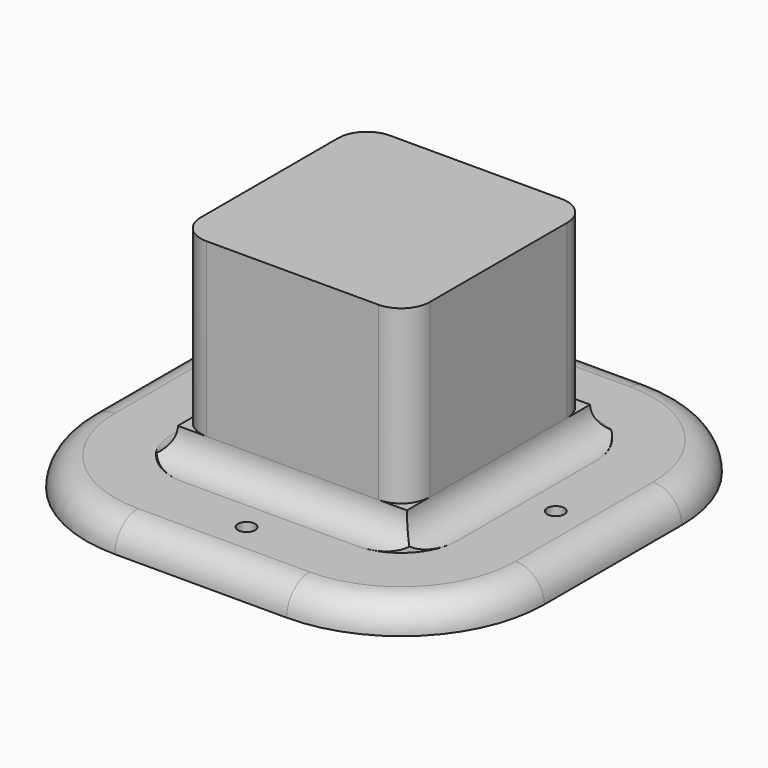
from build123d import *

# Parameters (mm, degrees)
F1_DEPTH  = 40
F0_R      = 1.5
F2_DEPTH  = 5
F3_R      = 4.99999
F4_DEPTH  = 10
F6_DEPTH  = 50
F7_DEPTH  = 5
F8_R      = 5
F9_DEPTH  = 50
F10_DEPTH = 5


# Not quite as in the source:
# - a fillet or chamfer is up to 0.001 mm smaller than in the source, because OpenCascade refuses the exact size


with BuildPart() as f1:
    # F0 (on Top) → F1 (new body)
    with BuildSketch(Plane.XY):
        with BuildLine():
            ThreePointArc((0, 5), (1.464466, 1.464466), (5, 0))
            Line((5, 0), (35, 0))
            ThreePointArc((35, 0), (38.535534, 1.464466), (40, 5))
            Line((40, 5), (40, 35))
            ThreePointArc((40, 35), (38.535534, 38.535534), (35, 40))
            Line((35, 40), (5, 40))
            ThreePointArc((5, 40), (1.464466, 38.535534), (0, 35))
            Line((0, 35), (0, 5))
        make_face()
    extrude(amount=F1_DEPTH)

    # F0 (on Top) → F2 (join)
    with BuildSketch(Plane.XY):
        with BuildLine():
            ThreePointArc((-20, 5), (-12.67767, -12.67767), (5, -20))
            Line((5, -20), (35, -20))
            ThreePointArc((35, -20), (52.67767, -12.67767), (60, 5))
            Line((60, 5), (60, 35))
            ThreePointArc((60, 35), (52.67767, 52.67767), (35, 60))
            Line((35, 60), (5, 60))
            ThreePointArc((5, 60), (-12.67767, 52.67767), (-20, 35))
            Line((-20, 35), (-20, 5))
        make_face()
        with Locations((20, -10)):
            Circle(F0_R, mode=Mode.SUBTRACT)
        with Locations((-10, 20)):
            Circle(F0_R, mode=Mode.SUBTRACT)
        with BuildLine():
            ThreePointArc((-5, 35), (-2.071068, 42.071068), (5, 45))
            Line((5, 45), (35, 45))
            ThreePointArc((35, 45), (42.071068, 42.071068), (45, 35))
            Line((45, 35), (45, 5))
            ThreePointArc((45, 5), (42.071068, -2.071068), (35, -5))
            Line((35, -5), (5, -5))
            ThreePointArc((5, -5), (-2.071068, -2.071068), (-5, 5))
            Line((-5, 5), (-5, 35))
        make_face(mode=Mode.SUBTRACT)
        with Locations((50, 20)):
            Circle(F0_R, mode=Mode.SUBTRACT)
        with Locations((20, 50)):
            Circle(F0_R, mode=Mode.SUBTRACT)
        with BuildLine():
            Line((35, 45), (5, 45))
            ThreePointArc((5, 45), (-2.071068, 42.071068), (-5, 35))
            Line((-5, 35), (-5, 5))
            ThreePointArc((-5, 5), (-2.071068, -2.071068), (5, -5))
            Line((5, -5), (35, -5))
            ThreePointArc((35, -5), (42.071068, -2.071068), (45, 5))
            Line((45, 5), (45, 35))
            ThreePointArc((45, 35), (42.071068, 42.071068), (35, 45))
        make_face()
        with BuildLine():
            Line((35, 0), (5, 0))
            ThreePointArc((5, 0), (1.464466, 1.464466), (0, 5))
            Line((0, 5), (0, 35))
            ThreePointArc((0, 35), (1.464466, 38.535534), (5, 40))
            Line((5, 40), (35, 40))
            ThreePointArc((35, 40), (38.535534, 38.535534), (40, 35))
            Line((40, 35), (40, 5))
            ThreePointArc((40, 5), (38.535534, 1.464466), (35, 0))
        make_face(mode=Mode.SUBTRACT)
    extrude(amount=F2_DEPTH)

    # F3 (radius 5 in the source; OpenCascade refuses exactly that, so slightly less here)
    f3_edges = [f1.edges().sort_by_distance(p)[0] for p in [
        (20, -20, 5),
        (0, 5, 22.5),
    ]]
    fillet(f3_edges, radius=F3_R)

    # F0 (on Top) → F4 (join)
    with BuildSketch(Plane.XY):
        with BuildLine():
            Line((35, 45), (5, 45))
            ThreePointArc((5, 45), (-2.071068, 42.071068), (-5, 35))
            Line((-5, 35), (-5, 5))
            ThreePointArc((-5, 5), (-2.071068, -2.071068), (5, -5))
            Line((5, -5), (35, -5))
            ThreePointArc((35, -5), (42.071068, -2.071068), (45, 5))
            Line((45, 5), (45, 35))
            ThreePointArc((45, 35), (42.071068, 42.071068), (35, 45))
        make_face()
        with BuildLine():
            Line((35, 0), (5, 0))
            ThreePointArc((5, 0), (1.464466, 1.464466), (0, 5))
            Line((0, 5), (0, 35))
            ThreePointArc((0, 35), (1.464466, 38.535534), (5, 40))
            Line((5, 40), (35, 40))
            ThreePointArc((35, 40), (38.535534, 38.535534), (40, 35))
            Line((40, 35), (40, 5))
            ThreePointArc((40, 5), (38.535534, 1.464466), (35, 0))
        make_face(mode=Mode.SUBTRACT)
    extrude(amount=F4_DEPTH)

    # F5 (on face) → F6 (cut)
    with BuildSketch(Plane.XZ.offset(5)):
        with BuildLine():
            ThreePointArc((50, 10), (41.464466, 13.535534), (45, 5))
            ThreePointArc((45, 5), (48.535534, 6.464466), (50, 10))
        make_face()
        with BuildLine():
            ThreePointArc((0, 10), (-8.535534, 13.535534), (-5, 5))
            ThreePointArc((-5, 5), (-1.464466, 6.464466), (0, 10))
        make_face()
    extrude(amount=-F6_DEPTH, mode=Mode.SUBTRACT)

    # F5 (on face) → F7 (cut)
    with BuildSketch(Plane.XZ.offset(5)):
        with BuildLine():
            ThreePointArc((50, 10), (41.464466, 13.535534), (45, 5))
            ThreePointArc((45, 5), (48.535534, 6.464466), (50, 10))
        make_face()
        with BuildLine():
            ThreePointArc((0, 10), (-8.535534, 13.535534), (-5, 5))
            ThreePointArc((-5, 5), (-1.464466, 6.464466), (0, 10))
        make_face()
    extrude(amount=F7_DEPTH, mode=Mode.SUBTRACT)

    # F8 (on face) → F9 (cut)
    with BuildSketch(Plane.YZ.offset(40)):
        with Locations((-5, 10)):
            Circle(F8_R)
        with Locations((45, 10)):
            Circle(F8_R)
    extrude(amount=-F9_DEPTH, mode=Mode.SUBTRACT)

    # F8 (on face) → F10 (cut)
    with BuildSketch(Plane.YZ.offset(40)):
        with Locations((-5, 10)):
            Circle(F8_R)
        with Locations((45, 10)):
            Circle(F8_R)
    extrude(amount=F10_DEPTH, mode=Mode.SUBTRACT)


solid = f1.part
